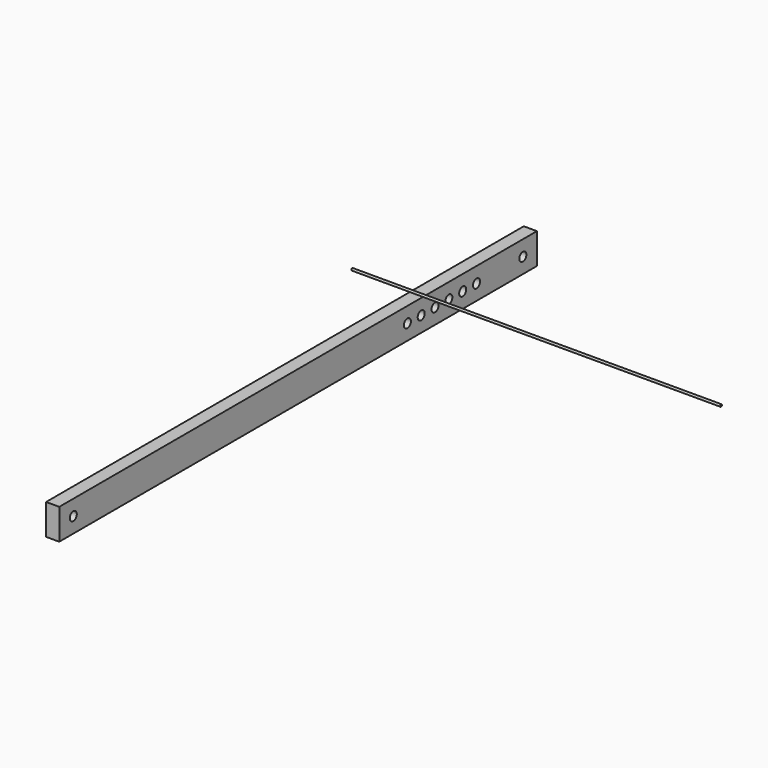
from build123d import *

# Parameters (mm, degrees)
F0_W     = 38.1
F0_H     = 88.9
F1_DEPTH = 1727.2
F3_D     = 25.4
F4_R     = 3.175
F5_DEPTH = 203.2
F6_DEPTH = 1066.8


# Not quite as in the source:
# - a feature names something its author has since deleted; it is built from what else it names


with BuildPart() as f1:
    # F0 (on Front) → F1 (new body)
    with BuildSketch(Plane.XZ):
        Rectangle(F0_W, F0_H)
    extrude(amount=F1_DEPTH)

    # F3 (through all)
    with Locations(Plane.YZ.offset(19.05)):
        with Locations((-468.4210526316, 0), (-418.4210526316, 0), (-368.4210526316, 0), (-318.4210526316, 0), (-50.8, 0), (-1676.4, 0), (-268.4210526316, 0), (-218.4210526316, 0)):
            Hole(F3_D / 2)


with BuildPart() as f5:
    # F4 (on face) → F5 (new body)
    with BuildSketch(Plane.YZ.offset(19.05)):
        with Locations((-1066.8073892593, 218.6309099197)):
            Circle(F4_R)
    extrude(amount=-F5_DEPTH)


with BuildPart() as f6:
    # F4 (on face) → F6 (new body)
    with BuildSketch(Plane.YZ.offset(19.05)):
        with Locations((-667.7466630936, 218.6309099197)):
            Circle(F4_R)
    extrude(amount=F6_DEPTH)


solid = Compound([f1.part, f6.part])
